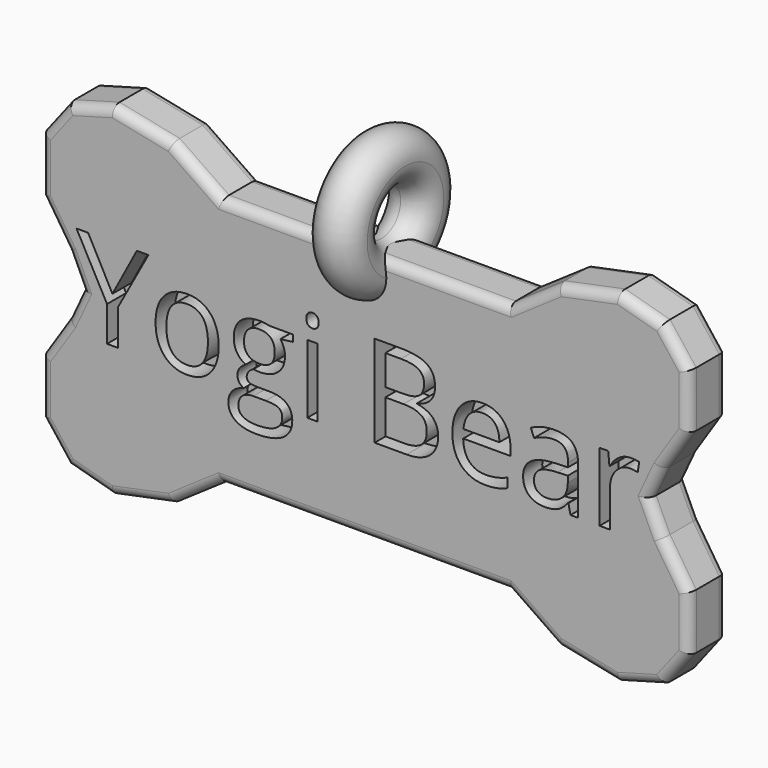
from build123d import *

# Parameters (mm, degrees)
F1_DEPTH     = 2.54
F2_R         = 0.508
F6_TEXT_SIZE = 6.8208668381
F7_DEPTH     = 1.27


# Not quite as in the source:
# - Text() gives the source's letters only with a copy of the font that has no kerning and outlines rounded to 1/6400 em; it was checked with that copy


with BuildPart() as f1:
    # F0 (on Front) → F1 (new body)
    with BuildSketch(Plane.XZ):
        Polygon((2.0103843274, 6.6693559441), (-5.6096156726, 6.6693559441), (-13.2296156726, 6.6693559441), (-15.8515510253, 8.4719367156), (-19.0470352022, 9.127420742), (-21.4231646474, 8.4719367156), (-22.8160668483, 6.6693559441), (-22.8160668483, 3.7196781265), (-21.4231646474, 1.5893559441), (-20.6857440637, 0), (-21.4231646474, -1.5893559441), (-22.8160668483, -3.7196781265), (-22.8160668483, -6.6693559441), (-21.4231646474, -8.4719367156), (-19.0470352022, -9.127420742), (-15.8515510253, -8.4719367156), (-13.2296156726, -6.6693559441), (-5.6096156726, -6.6693559441), (2.0103843274, -6.6693559441), (4.6323196802, -8.4719367156), (7.8278038571, -9.127420742), (10.2039333023, -8.4719367156), (11.5968355032, -6.6693559441), (11.5968355032, -3.7196781265), (10.2039333023, -1.5893559441), (9.4665127186, 0), (10.2039333023, 1.5893559441), (11.5968355032, 3.7196781265), (11.5968355032, 6.6693559441), (10.2039333023, 8.4719367156), (7.8278038571, 9.127420742), (4.6323196802, 8.4719367156), align=None)
    extrude(amount=F1_DEPTH)

    # F2
    f2_edges = [f1.edges().sort_by_distance(p)[0] for p in [
        (6.230062, -2.54, 8.799679),
        (3.321352, -2.54, 7.570646),
        (-5.609616, -2.54, 6.669356),
        (-14.540583, -2.54, 7.570646),
        (-17.449293, -2.54, 8.799679),
        (-20.2351, -2.54, 8.799679),
        (-22.119616, -2.54, 7.570646),
        (-22.816067, -2.54, 5.194517),
        (-22.119616, -2.54, 2.654517),
        (-21.054454, -2.54, 0.794678),
        (-21.054454, -2.54, -0.794678),
        (-22.119616, -2.54, -2.654517),
        (-22.816067, -2.54, -5.194517),
        (-22.119616, -2.54, -7.570646),
        (-20.2351, -2.54, -8.799679),
        (-17.449293, -2.54, -8.799679),
        (-14.540583, -2.54, -7.570646),
        (-5.609616, -2.54, -6.669356),
        (3.321352, -2.54, -7.570646),
        (6.230062, -2.54, -8.799679),
        (9.015869, -2.54, -8.799679),
        (10.900384, -2.54, -7.570646),
        (11.596836, -2.54, -5.194517),
        (10.900384, -2.54, -2.654517),
        (9.835223, -2.54, -0.794678),
        (9.835223, -2.54, 0.794678),
        (10.900384, -2.54, 2.654517),
        (11.596836, -2.54, 5.194517),
        (10.900384, -2.54, 7.570646),
        (9.015869, -2.54, 8.799679),
        (6.230062, 0, 8.799679),
        (3.321352, 0, 7.570646),
        (-5.609616, 0, 6.669356),
        (-14.540583, 0, 7.570646),
        (-17.449293, 0, 8.799679),
        (-20.2351, 0, 8.799679),
        (-22.119616, 0, 7.570646),
        (-22.816067, 0, 5.194517),
        (-22.119616, 0, 2.654517),
        (-21.054454, 0, 0.794678),
        (-21.054454, 0, -0.794678),
        (-22.119616, 0, -2.654517),
        (-22.816067, 0, -5.194517),
        (-22.119616, 0, -7.570646),
        (-20.2351, 0, -8.799679),
        (-17.449293, 0, -8.799679),
        (-14.540583, 0, -7.570646),
        (-5.609616, 0, -6.669356),
        (3.321352, 0, -7.570646),
        (6.230062, 0, -8.799679),
        (9.015869, 0, -8.799679),
        (10.900384, 0, -7.570646),
        (11.596836, 0, -5.194517),
        (10.900384, 0, -2.654517),
        (9.835223, 0, -0.794678),
        (9.835223, 0, 0.794678),
        (10.900384, 0, 2.654517),
        (11.596836, 0, 5.194517),
        (10.900384, 0, 7.570646),
        (9.015869, 0, 8.799679),
    ]]
    fillet(f2_edges, radius=F2_R)

    # F4 (on offset) → F5 (revolve)
    with BuildSketch(Plane.XZ.offset(1.27)):
        with BuildLine():
            ThreePointArc((-5.7404, 6.7623230782), (-6.6384256121, 4.5942974661), (-4.4704, 5.4923230782))
            ThreePointArc((-4.4704, 5.4923230782), (-4.8423743879, 6.3903486903), (-5.7404, 6.7623230782))
        make_face()
    revolve(axis=Axis((-2.6754314768, -1.27, 8.0323230782), (1, 0, 0)))

    # F6 (on face) → F7 (cut)
    with BuildSketch(Plane.XZ.offset(2.54)):
        with Locations((-20.9349915385, -2.061081701)):
            Text('Yogi Bear', F6_TEXT_SIZE, font='Open Sans', text_align=(TextAlign.LEFT, TextAlign.BOTTOM))
    extrude(amount=-F7_DEPTH, mode=Mode.SUBTRACT)


solid = f1.part
